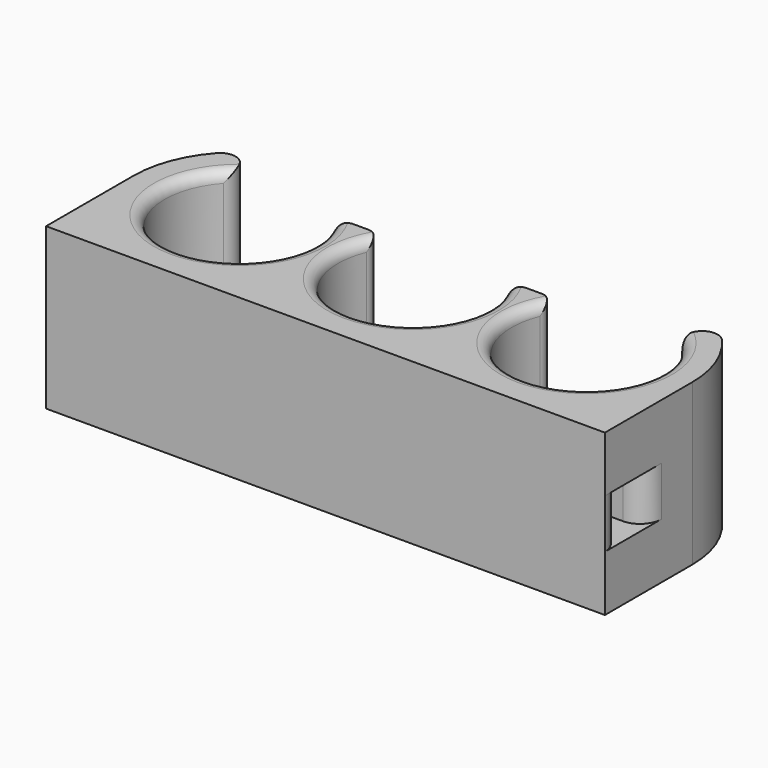
from build123d import *

# Parameters (mm, degrees)
F1_DEPTH     = 19.05
F3_W         = 3.302
F3_H         = 5.842
F4_DEPTH     = 66.2855144291
F5_R         = 2.53999
F6_T2_ANGLE  = 285.0642711804
F6_T4_ANGLE  = 265.7478080458
F6_T6_ANGLE  = 285.2154653986
F6_T8_ANGLE  = 285.2154653986
F6_T10_ANGLE = 265.7478080458
F6_T12_ANGLE = 285.0642711804


# Not quite as in the source:
# - a fillet or chamfer that OpenCascade refuses, or shapes differently, is made with other operations: its cross-section is extruded or revolved along the edge and cut away or added
# - a fillet or chamfer is up to 0.001 mm smaller than in the source, because OpenCascade refuses the exact size


with BuildPart() as f1:
    # F0 (on Top) → F1 (new body)
    with BuildSketch(Plane.XY):
        with BuildLine():
            Line((-12.5682572145, -12.9684638232), (53.7162572145, -12.9684638232))
            Line((53.7162572145, -12.9684638232), (53.7162572145, 0))
            ThreePointArc((53.7162572145, 0), (52.8949248233, 4.4688753179), (50.5382753725, 8.35367092))
            ThreePointArc((50.5382753725, 8.35367092), (47.9416524269, 8.5053660876), (47.7899572593, 5.908743142))
            ThreePointArc((47.7899572593, 5.908743142), (42.6379125223, -8.7640745335), (32.9266056139, 3.3819396952))
            ThreePointArc((32.9266056139, 3.3819396952), (32.807201494, 4.5719455748), (31.7520964907, 5.1350838967))
            Line((31.7520964907, 5.1350838967), (29.9701016635, 5.1350838967))
            ThreePointArc((29.9701016635, 5.1350838967), (28.9149992826, 4.5719494891), (28.7955889556, 3.3819484096))
            ThreePointArc((28.7955889556, 3.3819484096), (20.574, -8.89), (12.3524110444, 3.3819484096))
            ThreePointArc((12.3524110444, 3.3819484096), (12.2330007174, 4.5719494891), (11.1778983365, 5.1350838967))
            Line((11.1778983365, 5.1350838967), (9.3961016635, 5.1350838967))
            ThreePointArc((9.3961016635, 5.1350838967), (8.3409992826, 4.5719494891), (8.2215889556, 3.3819484096))
            ThreePointArc((8.2215889556, 3.3819484096), (-1.501623816, -8.7622614612), (-6.6263626723, 5.9265013064))
            ThreePointArc((-6.6263626723, 5.9265013064), (-6.8025064605, 8.5131919049), (-9.3902753725, 8.35367092))
            ThreePointArc((-9.3902753725, 8.35367092), (-11.7469248233, 4.4688753179), (-12.5682572145, 0))
            Line((-12.5682572145, 0), (-12.5682572145, -12.9684638232))
        make_face()
    extrude(amount=F1_DEPTH)

    # F3 (on offset) → F4 (cut, through all)
    with BuildSketch(Plane.YZ.offset(53.7162572145)):
        with Locations((-8.7774638232, 9.525)):
            Rectangle(F3_W, F3_H)
    extrude(amount=-F4_DEPTH, mode=Mode.SUBTRACT)

    # F5 (radius 2.54 in the source; OpenCascade refuses exactly that, so slightly less here)
    f5_edges = [f1.edges().sort_by_distance(p)[0] for p in [
        (53.716257, -10.428464, 9.525),
        (53.716257, -7.126464, 9.525),
        (-12.568257, -7.126464, 9.525),
        (-12.568257, -10.428464, 9.525),
    ]]
    fillet(f5_edges, radius=F5_R)

    # F6: fillet of radius 1.27 on 6 edges, made by hand

    # F6_s1 → F6_t2 (revolve, cut)
    with BuildSketch(Plane(origin=(32.1859589237, -16.9838713477, 0), x_dir=(0, 0, 1), z_dir=(-0.8844206226, 0.4666906494, 0))):
        with BuildLine():
            ThreePointArc((1.27, 28.0932035867), (0.3719743879, 28.4651779746), (0, 29.3632035867))
            Line((0, 29.3632035867), (0, 28.0932035867))
            Line((0, 28.0932035867), (1.27, 28.0932035867))
        make_face()
    revolve(axis=Axis((41.148, 0, 0), (0, 0, -1)), revolution_arc=F6_T2_ANGLE, mode=Mode.SUBTRACT)

    # F6_s3 → F6_t4 (revolve, cut)
    with BuildSketch(Plane(origin=(9.5242534962, -10.2586834814, 0), x_dir=(0, 0, 1), z_dir=(-0.6803871538, 0.7328528644, 0))):
        with BuildLine():
            ThreePointArc((1.27, 23.9677148325), (0.3719743879, 24.3396892203), (0, 25.2377148325))
            Line((0, 25.2377148325), (0, 23.9677148325))
            Line((0, 23.9677148325), (1.27, 23.9677148325))
        make_face()
    revolve(axis=Axis((20.574, 0, 0), (0, 0, -1)), revolution_arc=F6_T4_ANGLE, mode=Mode.SUBTRACT)

    # F6_s5 → F6_t6 (revolve, cut)
    with BuildSketch(Plane(origin=(0, 0, 0), x_dir=(0, 0, 1), z_dir=(-0.6805059381, 0.7327425661, 0))):
        with BuildLine():
            ThreePointArc((1.27, 8.89), (0.3719743879, 9.2619743879), (0, 10.16))
            Line((0, 10.16), (0, 8.89))
            Line((0, 8.89), (1.27, 8.89))
        make_face()
    revolve(axis=Axis((0, 0, 0), (0, 0, -1)), revolution_arc=F6_T6_ANGLE, mode=Mode.SUBTRACT)

    # F6_s7 → F6_t8 (revolve, cut)
    with BuildSketch(Plane(origin=(0, 0, 0), x_dir=(0, 0, 1), z_dir=(-0.6805059381, 0.7327425661, 0))):
        with BuildLine():
            ThreePointArc((17.78, 8.89), (18.6780256121, 9.2619743879), (19.05, 10.16))
            Line((19.05, 10.16), (19.05, 8.89))
            Line((19.05, 8.89), (17.78, 8.89))
        make_face()
    revolve(axis=Axis((0, 0, 19.05), (0, 0, -1)), revolution_arc=F6_T8_ANGLE, mode=Mode.SUBTRACT)

    # F6_s9 → F6_t10 (revolve, cut)
    with BuildSketch(Plane(origin=(9.5242534962, -10.2586834814, 0), x_dir=(0, 0, 1), z_dir=(-0.6803871538, 0.7328528644, 0))):
        with BuildLine():
            ThreePointArc((17.78, 23.9677148325), (18.6780256121, 24.3396892203), (19.05, 25.2377148325))
            Line((19.05, 25.2377148325), (19.05, 23.9677148325))
            Line((19.05, 23.9677148325), (17.78, 23.9677148325))
        make_face()
    revolve(axis=Axis((20.574, 0, 19.05), (0, 0, -1)), revolution_arc=F6_T10_ANGLE, mode=Mode.SUBTRACT)

    # F6_s11 → F6_t12 (revolve, cut)
    with BuildSketch(Plane(origin=(32.1859589237, -16.9838713477, 0), x_dir=(0, 0, 1), z_dir=(-0.8844206226, 0.4666906494, 0))):
        with BuildLine():
            ThreePointArc((17.78, 28.0932035867), (18.6780256121, 28.4651779746), (19.05, 29.3632035867))
            Line((19.05, 29.3632035867), (19.05, 28.0932035867))
            Line((19.05, 28.0932035867), (17.78, 28.0932035867))
        make_face()
    revolve(axis=Axis((41.148, 0, 19.05), (0, 0, -1)), revolution_arc=F6_T12_ANGLE, mode=Mode.SUBTRACT)


solid = f1.part
